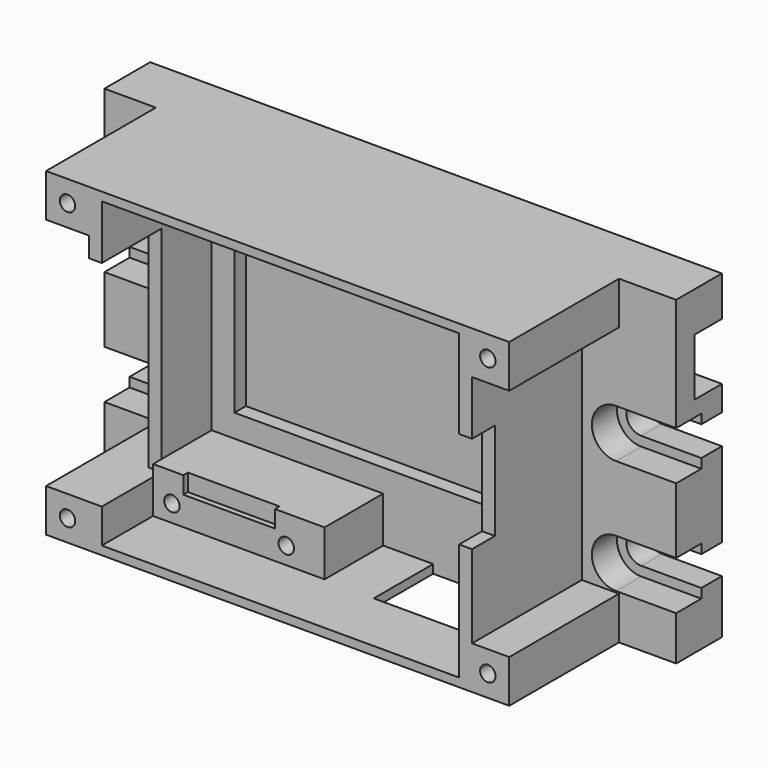
from build123d import *

# Parameters (mm, degrees)
F1_DEPTH  = 12
F3_DEPTH  = 5
F4_W      = 100
F4_H      = 56
F5_DEPTH  = 2
F6_W      = 130
F6_H      = 5
F7_DEPTH  = 12.001
F9_DEPTH  = 10.001
F11_DEPTH = 5.5
F12_W     = 67
F12_H     = 56
F12_W_2   = 62.5
F12_H_2   = 53
F13_DEPTH = 24
F14_W     = 30
F14_H     = 8
F15_DEPTH = 12.8
F16_W     = 13
F16_H     = 37.5
F17_DEPTH = 2.25
F18_W     = 20
F18_H     = 13
F19_DEPTH = 1.5
F21_D     = 2.7
F21_DEPTH = 12
F21_TIP   = 0.8111618357
F22_W     = 50.5
F22_H     = 38
F23_DEPTH = 2.5
F24_W     = 6.5
F24_H     = 7.5
F24_W_2   = 1
F24_W_3   = 7.5
F25_DEPTH = 24
F27_D     = 2.7
F27_DEPTH = 12
F27_TIP   = 0.8111618357
F28_W     = 5
F28_H     = 17
F29_DEPTH = 2.25
F30_W     = 15
F30_H     = 10
F31_DEPTH = 6
F32_W     = 16
F32_H     = 3
F33_DEPTH = 1


# Not quite as in the source:
# - a feature names something its author has since deleted; it is built from what else it names


with BuildPart() as f1:
    # F0 (on Front) → F1 (new body)
    with BuildSketch(Plane.XZ):
        Polygon((-65, 5), (-65, 0), (65, 0), (65, 5), (50, 5), (50, 61), (-50, 61), (-50, 5), align=None)
    extrude(amount=F1_DEPTH)

    # F2 (on face) → F3 (cut, through all)
    with BuildSketch(Plane(origin=(0, 0, 0), x_dir=(1, 0, 0), z_dir=(0, 0, -1))):
        with BuildLine():
            Line((-65, 2.65), (-63, 2.65))
            ThreePointArc((-63, 2.65), (-59.65, 6), (-63, 9.35))
            Line((-63, 9.35), (-65, 9.35))
            Line((-65, 9.35), (-65, 2.65))
        make_face()
        with BuildLine():
            Line((65, 9.35), (63, 9.35))
            ThreePointArc((63, 9.35), (59.65, 6), (63, 2.65))
            Line((63, 2.65), (65, 2.65))
            Line((65, 2.65), (65, 9.35))
        make_face()
    extrude(amount=-F3_DEPTH, mode=Mode.SUBTRACT)

    # F4 (on face) → F5 (cut)
    with BuildSketch(Plane(origin=(0, 0, 0), x_dir=(-1, 0, 0), z_dir=(0, 1, 0))):
        with Locations((0, 33)):
            Rectangle(F4_W, F4_H)
    extrude(amount=-F5_DEPTH, mode=Mode.SUBTRACT)

    # F6 (on face) → F7 (cut, through all)
    with BuildSketch(Plane(origin=(0, 0, 0), x_dir=(-1, 0, 0), z_dir=(0, 1, 0))):
        with Locations((0, 2.5)):
            Rectangle(F6_W, F6_H)
    extrude(amount=-F7_DEPTH, mode=Mode.SUBTRACT)

    # F8 (on face) → F9 (cut, through all)
    with BuildSketch(Plane.XZ.offset(12)):
        with BuildLine():
            ThreePointArc((-39.5, 34.4), (-36.9, 37), (-39.5, 39.6))
            Line((-39.5, 39.6), (-50, 39.6))
            Line((-50, 39.6), (-50, 34.4))
            Line((-50, 34.4), (-39.5, 34.4))
        make_face()
        with BuildLine():
            Line((-39.5, 19.6), (-50, 19.6))
            Line((-50, 19.6), (-50, 14.4))
            Line((-50, 14.4), (-39.5, 14.4))
            ThreePointArc((-39.5, 14.4), (-36.9, 17), (-39.5, 19.6))
        make_face()
        with BuildLine():
            Line((50, 39.6), (39.5, 39.6))
            ThreePointArc((39.5, 39.6), (36.9, 37), (39.5, 34.4))
            Line((39.5, 34.4), (50, 34.4))
            Line((50, 34.4), (50, 39.6))
        make_face()
        with BuildLine():
            Line((50, 14.4), (50, 19.6))
            Line((50, 19.6), (39.5, 19.6))
            ThreePointArc((39.5, 19.6), (36.9, 17), (39.5, 14.4))
            Line((39.5, 14.4), (50, 14.4))
        make_face()
    extrude(amount=-F9_DEPTH, mode=Mode.SUBTRACT)

    # F10 (on face) → F11 (cut)
    with BuildSketch(Plane.XZ.offset(12)):
        with BuildLine():
            Line((-50, 32.75), (-39.5, 32.75))
            ThreePointArc((-39.5, 32.75), (-35.25, 37), (-39.5, 41.25))
            Line((-39.5, 41.25), (-50, 41.25))
            Line((-50, 41.25), (-50, 39.6))
            Line((-50, 39.6), (-39.5, 39.6))
            ThreePointArc((-39.5, 39.6), (-36.9, 37), (-39.5, 34.4))
            Line((-39.5, 34.4), (-50, 34.4))
            Line((-50, 34.4), (-50, 32.75))
        make_face()
        with BuildLine():
            Line((-39.5, 21.25), (-50, 21.25))
            Line((-50, 21.25), (-50, 19.6))
            Line((-50, 19.6), (-39.5, 19.6))
            ThreePointArc((-39.5, 19.6), (-36.9, 17), (-39.5, 14.4))
            Line((-39.5, 14.4), (-50, 14.4))
            Line((-50, 14.4), (-50, 12.75))
            Line((-50, 12.75), (-39.5, 12.75))
            ThreePointArc((-39.5, 12.75), (-35.25, 17), (-39.5, 21.25))
        make_face()
        with BuildLine():
            Line((50, 39.6), (50, 41.25))
            Line((50, 41.25), (39.5, 41.25))
            ThreePointArc((39.5, 41.25), (35.25, 37), (39.5, 32.75))
            Line((39.5, 32.75), (50, 32.75))
            Line((50, 32.75), (50, 34.4))
            Line((50, 34.4), (39.5, 34.4))
            ThreePointArc((39.5, 34.4), (36.9, 37), (39.5, 39.6))
            Line((39.5, 39.6), (50, 39.6))
        make_face()
        with BuildLine():
            Line((39.5, 12.75), (50, 12.75))
            Line((50, 12.75), (50, 14.4))
            Line((50, 14.4), (39.5, 14.4))
            ThreePointArc((39.5, 14.4), (36.9, 17), (39.5, 19.6))
            Line((39.5, 19.6), (50, 19.6))
            Line((50, 19.6), (50, 21.25))
            Line((50, 21.25), (39.5, 21.25))
            ThreePointArc((39.5, 21.25), (35.25, 17), (39.5, 12.75))
        make_face()
    extrude(amount=-F11_DEPTH, mode=Mode.SUBTRACT)

    # F12 (on face) → F13 (join)
    with BuildSketch(Plane.XZ.offset(12)):
        with Locations((0, 33)):
            Rectangle(F12_W, F12_H)
        with Locations((0, 33)):
            Rectangle(F12_W_2, F12_H_2, mode=Mode.SUBTRACT)
    extrude(amount=F13_DEPTH)

    # F14 (on face) → F15 (join)
    with BuildSketch(Plane.XZ.offset(12)):
        with Locations((-16.25, 10.5)):
            Rectangle(F14_W, F14_H)
    extrude(amount=F15_DEPTH)

    # F16 (on face) → F17 (cut, through all)
    with BuildSketch(Plane(origin=(-33.5, 0, 0), x_dir=(0, -1, 0), z_dir=(-1, 0, 0))):
        with Locations((29.5, 31.25)):
            Rectangle(F16_W, F16_H)
    extrude(amount=-F17_DEPTH, mode=Mode.SUBTRACT)

    # F18 (on face) → F19 (cut, through all)
    with BuildSketch(Plane(origin=(0, 0, 5), x_dir=(1, 0, 0), z_dir=(0, 0, -1))):
        with Locations((17.5, 18.5)):
            Rectangle(F18_W, F18_H)
    extrude(amount=-F19_DEPTH, mode=Mode.SUBTRACT)

    # F21
    with Locations(Plane.XZ.offset(24.8)):
        with Locations((-27.95, 9.5), (-7.95, 9.5)):
            Hole(F21_D / 2, depth=F21_DEPTH)
            with Locations((0, 0, -(F21_DEPTH + F21_TIP / 2))):  # 118° drill point
                Cone(0, F21_D / 2, F21_TIP, mode=Mode.SUBTRACT)

    # F22 (on face) → F23 (cut)
    with BuildSketch(Plane.XZ.offset(12)):
        with Locations((-2, 37.5)):
            Rectangle(F22_W, F22_H)
    extrude(amount=-F23_DEPTH, mode=Mode.SUBTRACT)

    # F24 (on face) → F25 (join, through all)
    with BuildSketch(Plane.XZ.offset(12)):
        with Locations((36.75, 57.25)):
            Rectangle(F24_W, F24_H)
        with Locations((33, 57.25)):
            Rectangle(F24_W_2, F24_H)
        with Locations((36.75, 8.75)):
            Rectangle(F24_W, F24_H)
        with Locations((33, 8.75)):
            Rectangle(F24_W_2, F24_H)
        with Locations((-37.25, 8.75)):
            Rectangle(F24_W_3, F24_H)
        with Locations((-37.25, 57.25)):
            Rectangle(F24_W_3, F24_H)
    extrude(amount=F25_DEPTH)

    # F27
    with Locations(Plane.XZ.offset(36)):
        with Locations((36.25, 57.25), (36.25, 8.75), (-37.25, 8.75), (-37.25, 57.25)):
            Hole(F27_D / 2, depth=F27_DEPTH)
            with Locations((0, 0, -(F27_DEPTH + F27_TIP / 2))):  # 118° drill point
                Cone(0, F27_D / 2, F27_TIP, mode=Mode.SUBTRACT)

    # F28 (on face) → F29 (cut, through all)
    with BuildSketch(Plane.YZ.offset(33.5)):
        with Locations((-33.5, 35.5)):
            Rectangle(F28_W, F28_H)
    extrude(amount=-F29_DEPTH, mode=Mode.SUBTRACT)

    # F30 (on face) → F31 (cut)
    with BuildSketch(Plane(origin=(0, -2, 0), x_dir=(-1, 0, 0), z_dir=(0, 1, 0))):
        with Locations((-42.5, 49)):
            Rectangle(F30_W, F30_H)
    extrude(amount=-F31_DEPTH, mode=Mode.SUBTRACT)

    # F32 (on face) → F33 (cut)
    with BuildSketch(Plane.XZ.offset(24.8)):
        with Locations((-17.95, 13)):
            Rectangle(F32_W, F32_H)
    extrude(amount=-F33_DEPTH, mode=Mode.SUBTRACT)


solid = f1.part
